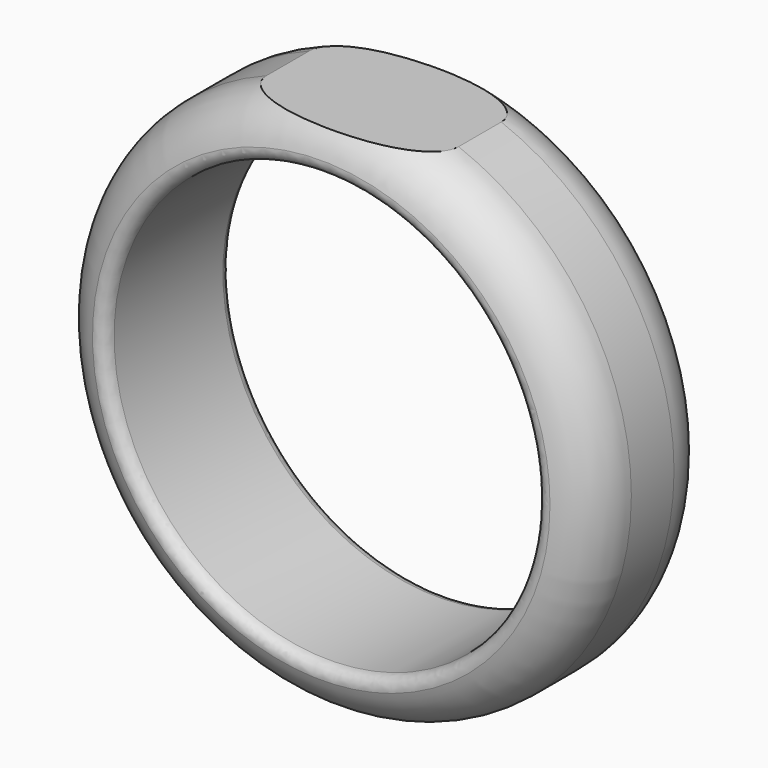
from build123d import *

# Parameters (mm, degrees)
F0_R     = 127.9602052378
F1_DEPTH = 76.2
F2_R     = 25.4
F3_DEPTH = 101.6
F4_R     = 5.08
F5_W     = 206.9260179996
F5_H     = 31.6136926413
F6_DEPTH = 101.6


with BuildPart() as f1:
    # F0 (on Front) → F1 (new body)
    with BuildSketch(Plane.XZ):
        Circle(F0_R)
    extrude(amount=F1_DEPTH)

    # F2
    f2_edges = [f1.edges().sort_by_distance(p)[0] for p in [
        (-127.960205, -76.2, 0),
        (-127.960205, 0, 0),
    ]]
    fillet(f2_edges, radius=F2_R)

    # F3 (cut): a face of the model
    f3_faces = [f1.faces().sort_by_distance(p)[0] for p in [
        (0, -76.2, 0),
    ]]
    extrude(f3_faces, amount=-F3_DEPTH, mode=Mode.SUBTRACT)

    # F4
    f4_edges = [f1.edges().sort_by_distance(p)[0] for p in [
        (127.960205, -38.1, 0),
        (-127.960205, -25.4, 0),
        (-127.960205, -50.8, 0),
        (-102.560205, 0, 0),
        (-102.560205, -76.2, 0),
    ]]
    fillet(f4_edges, radius=F4_R)

    # F5 (on Front) → F6 (cut)
    with BuildSketch(Plane.XZ):
        with Locations((3.8319602609, 135.3162005544)):
            Rectangle(F5_W, F5_H)
    extrude(amount=F6_DEPTH, mode=Mode.SUBTRACT)


solid = f1.part
